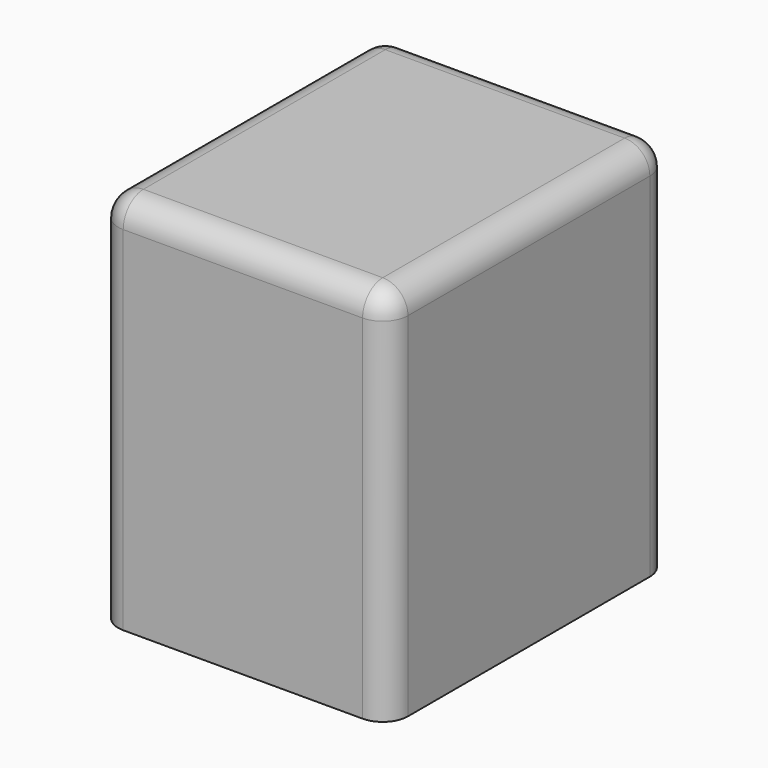
from build123d import *

# Parameters (mm, degrees)
F0_W     = 23
F0_H     = 28
F1_DEPTH = 30
F2_R     = 2
F3_R     = 2
F4_R     = 2
F5_R     = 2
F6_R     = 2
F7_T     = 2
F8_R     = 2


# Not quite as in the source:
# - a feature of the source that left no trace in its solid (it failed there, or was rolled back) is left out
# - a shell that OpenCascade refuses in one call is made with other operations: the cavity is built on its own and cut out


with BuildPart() as f1:
    # F0 (on Top) → F1 (new body)
    with BuildSketch(Plane.XY):
        with Locations((-41.8064879576, 45.8027429283)):
            Rectangle(F0_W, F0_H)
    extrude(amount=F1_DEPTH)

    # F2
    f2_edges = [f1.edges().sort_by_distance(p)[0] for p in [
        (-30.306488, 31.802743, 15),
    ]]
    fillet(f2_edges, radius=F2_R)

    # F3
    f3_edges = [f1.edges().sort_by_distance(p)[0] for p in [
        (-30.306488, 59.802743, 15),
    ]]
    fillet(f3_edges, radius=F3_R)

    # F4
    f4_edges = [f1.edges().sort_by_distance(p)[0] for p in [
        (-53.306488, 31.802743, 15),
    ]]
    fillet(f4_edges, radius=F4_R)

    # F5
    f5_edges = [f1.edges().sort_by_distance(p)[0] for p in [
        (-53.306488, 59.802743, 15),
    ]]
    fillet(f5_edges, radius=F5_R)

    # F6
    f6_edges = [f1.edges().sort_by_distance(p)[0] for p in [
        (-41.806488, 31.802743, 30),
    ]]
    fillet(f6_edges, radius=F6_R)

    # F7: shell of thickness 2, made by hand


with BuildPart() as f7_core1:
    # F7_t2: copy of F1
    add(f1.part)

    # the walls: a layer under each face that stays
    f7_faces = [f7_core1.faces().sort_by_distance(p)[0] for p in [
        (-53.3064879576, 45.8027429283, 14),
        (-41.8064879576, 59.8027429283, 14),
        (-41.8064879576, 45.8027429283, 30),
        (-41.8064879576, 31.8027429283, 14),
        (-30.3064879576, 45.8027429283, 14),
    ]]
    thicken(f7_faces, amount=-F7_T, mode=Mode.SUBTRACT)


with BuildPart() as f1_1:
    add(f1.part)

    # what is left inside the walls is the cavity
    f7_cavity = [f7_core1.part.solids().sort_by_distance(p)[0] for p in [
        (-51.286488, 45.802743, 18.666667),
    ]]
    add(f7_cavity, mode=Mode.SUBTRACT)

    # F8
    f8_edges = [f1_1.edges().sort_by_distance(p)[0] for p in [
        (-51.306488, 57.802743, 14),
        (-51.306488, 33.802743, 14),
        (-32.306488, 33.802743, 14),
        (-32.306488, 57.802743, 14),
    ]]
    fillet(f8_edges, radius=F8_R)


solid = f1_1.part
